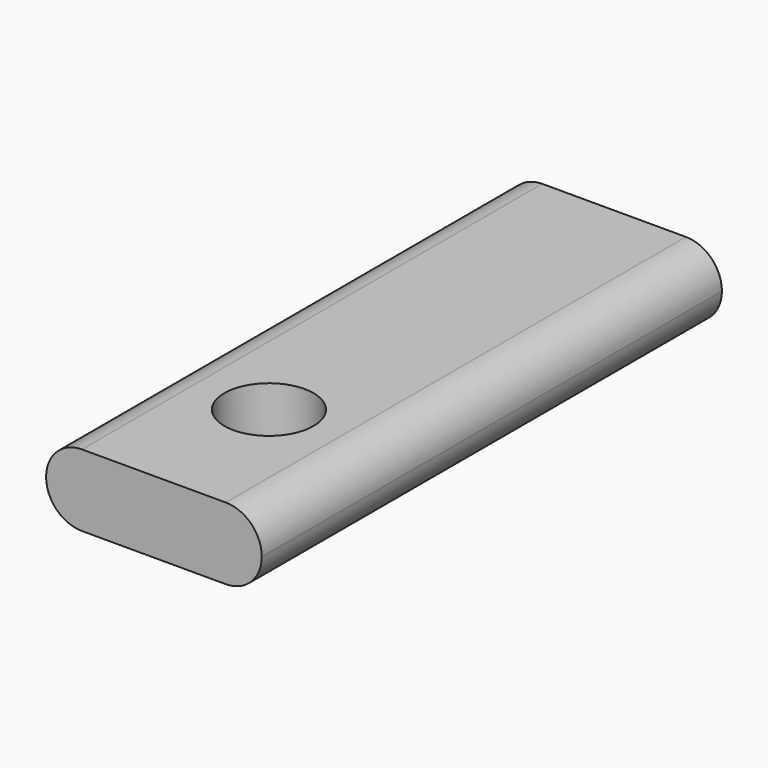
from build123d import *

# Parameters (mm, degrees)
F0_W     = 38.10014986
F0_H     = 12.7
F1_DEPTH = 50.8
F2_R     = 6.34999
F3_R     = 7.874
F4_DEPTH = 12.701


# Not quite as in the source:
# - a fillet or chamfer is up to 0.001 mm smaller than in the source, because OpenCascade refuses the exact size


with BuildPart() as f1:
    # F0 (on Front) → F1 (new body, symmetric)
    with BuildSketch(Plane.XZ):
        Rectangle(F0_W, F0_H)
    extrude(amount=F1_DEPTH, both=True)

    # F2 (radius 6.35 in the source; OpenCascade refuses exactly that, so slightly less here)
    f2_edges = [f1.edges().sort_by_distance(p)[0] for p in [
        (-19.050075, 0, 6.35),
        (19.050075, 0, 6.35),
        (19.050075, 0, -6.35),
        (-19.050075, 0, -6.35),
    ]]
    fillet(f2_edges, radius=F2_R)

    # F3 (on face) → F4 (cut, through all)
    with BuildSketch(Plane.XY.offset(6.35)):
        with Locations((0, -25.4)):
            Circle(F3_R)
    extrude(amount=-F4_DEPTH, mode=Mode.SUBTRACT)


solid = f1.part
